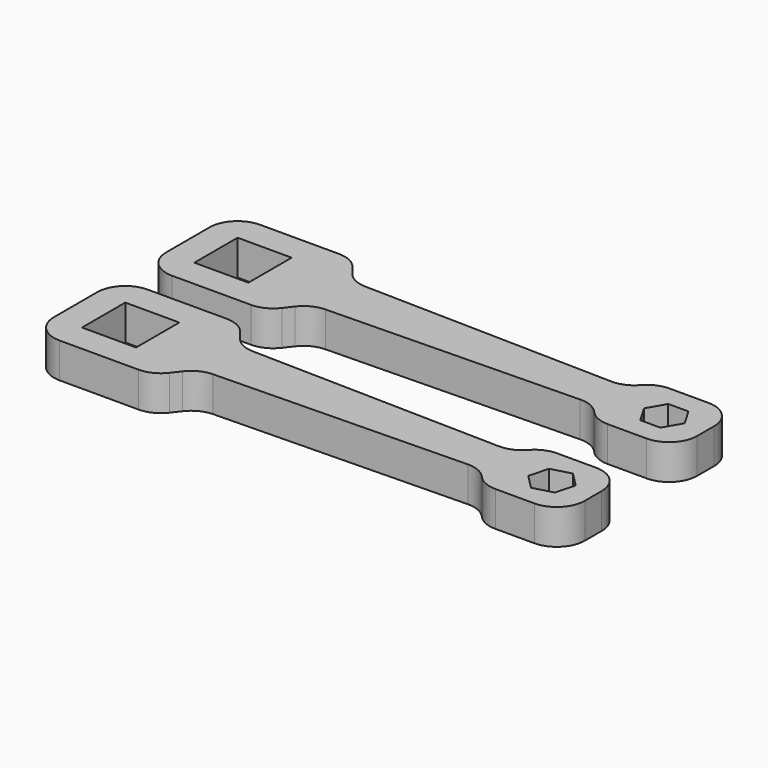
from build123d import *

# Parameters (mm, degrees)
F0_W         = 9.779
F0_H         = 9.779
F1_DEPTH     = 6.35
F2_R         = 5.08
F7_DEPTH     = 6.35
F9_DEPTH     = 25.4
F10_T1_DEPTH = 6.35
F11_R        = 5.08
F12_T1_DEPTH = 6.35
F13_R        = 5.08


# Not quite as in the source:
# - a fillet or chamfer that OpenCascade refuses, or shapes differently, is made with other operations: its cross-section is extruded or revolved along the edge and cut away or added


with BuildPart() as f1:
    # F0 (on Top) → F1 (new body)
    with BuildSketch(Plane.XY):
        Polygon((-20.7929461649, 4.5447559669), (-24.958435446, 9.9695), (-46.8228371047, 9.9695), (-46.8228371047, -9.9695), (-24.958435446, -9.9695), (-20.7929461649, -4.5447559669), (31.870488686, -3.4241478445), (31.870488686, -6.985), (46.8228371047, -6.985), (46.8228371047, 6.985), (31.870488686, 6.985), (31.870488686, 3.4241478445), align=None)
        with Locations((-36.8533371047, 0)):
            Rectangle(F0_W, F0_H, mode=Mode.SUBTRACT)
        Polygon((41.17975, -3.175), (37.5135757906, -3.175), (35.680488686, 0), (37.5135757906, 3.175), (41.17975, 3.175), (43.0128371047, 0), align=None, mode=Mode.SUBTRACT)
    extrude(amount=F1_DEPTH)

    # F2
    f2_edges = [f1.edges().sort_by_distance(p)[0] for p in [
        (-46.822837, -9.9695, 3.175),
        (-46.822837, 9.9695, 3.175),
        (46.822837, 6.985, 3.175),
        (-20.792946, 4.544756, 3.175),
        (-24.958435, 9.9695, 3.175),
        (-24.958435, -9.9695, 3.175),
        (-20.792946, -4.544756, 3.175),
        (46.822837, -6.985, 3.175),
    ]]
    fillet(f2_edges, radius=F2_R)


with BuildPart() as f5_1:
    # F5: copy of F1
    add(f1.part.moved(Location((0, -25.4, 0))))

    # F6 (on Top) → F7 (join, through all)
    with BuildSketch(Plane.XY):
        Polygon((41.17975, -22.225), (37.5135757906, -22.225), (35.680488686, -25.4), (37.5135757906, -28.575), (41.17975, -28.575), (43.0128371047, -25.4), align=None)
    extrude(amount=F7_DEPTH)

    # F8 (on face) → F9 (cut)
    with BuildSketch(Plane.XY.offset(6.35)):
        Polygon((40.2955386034, -21.8587476475), (36.7542862509, -22.8076233556), (35.8054105428, -26.348875708), (38.3977871873, -28.9412523525), (41.9390395398, -27.9923766444), (42.8879152478, -24.451124292), align=None)
    extrude(amount=-F9_DEPTH, mode=Mode.SUBTRACT)

    # F12: fillet of radius 5.08 on 2 edges, made by hand

    # F12_s2 → F12_t1 (join)
    with BuildSketch(Plane.XY):
        with BuildLine():
            ThreePointArc((31.870488686, -32.385), (29.9759334624, -29.8503125373), (26.9485679852, -28.9288797962))
            Line((26.9485679852, -28.9288797962), (31.870488686, -28.8241478445))
            Line((31.870488686, -28.8241478445), (31.870488686, -32.385))
        make_face()
        with BuildLine():
            ThreePointArc((31.870488686, -18.415), (29.9759334624, -20.9496874627), (26.9485679852, -21.8711202038))
            Line((26.9485679852, -21.8711202038), (31.870488686, -21.9758521555))
            Line((31.870488686, -21.9758521555), (31.870488686, -18.415))
        make_face()
    extrude(amount=F12_T1_DEPTH)

    # F13
    f13_edges = [f5_1.edges().sort_by_distance(p)[0] for p in [
        (31.870489, -18.415, 3.175),
        (31.870489, -32.385, 3.175),
    ]]
    fillet(f13_edges, radius=F13_R)


with BuildPart() as f1_1:
    add(f1.part)

    # F10: fillet of radius 5.08 on 2 edges, made by hand

    # F10_s2 → F10_t1 (join)
    with BuildSketch(Plane.XY):
        with BuildLine():
            ThreePointArc((31.870488686, 6.985), (29.9759334624, 4.4503125373), (26.9485679852, 3.5288797962))
            Line((26.9485679852, 3.5288797962), (31.870488686, 3.4241478445))
            Line((31.870488686, 3.4241478445), (31.870488686, 6.985))
        make_face()
        with BuildLine():
            ThreePointArc((31.870488686, -6.985), (29.9759334624, -4.4503125373), (26.9485679852, -3.5288797962))
            Line((26.9485679852, -3.5288797962), (31.870488686, -3.4241478445))
            Line((31.870488686, -3.4241478445), (31.870488686, -6.985))
        make_face()
    extrude(amount=F10_T1_DEPTH)

    # F11
    f11_edges = [f1_1.edges().sort_by_distance(p)[0] for p in [
        (31.870489, -6.985, 3.175),
        (31.870489, 6.985, 3.175),
    ]]
    fillet(f11_edges, radius=F11_R)


solid = Compound([f5_1.part, f1_1.part])
